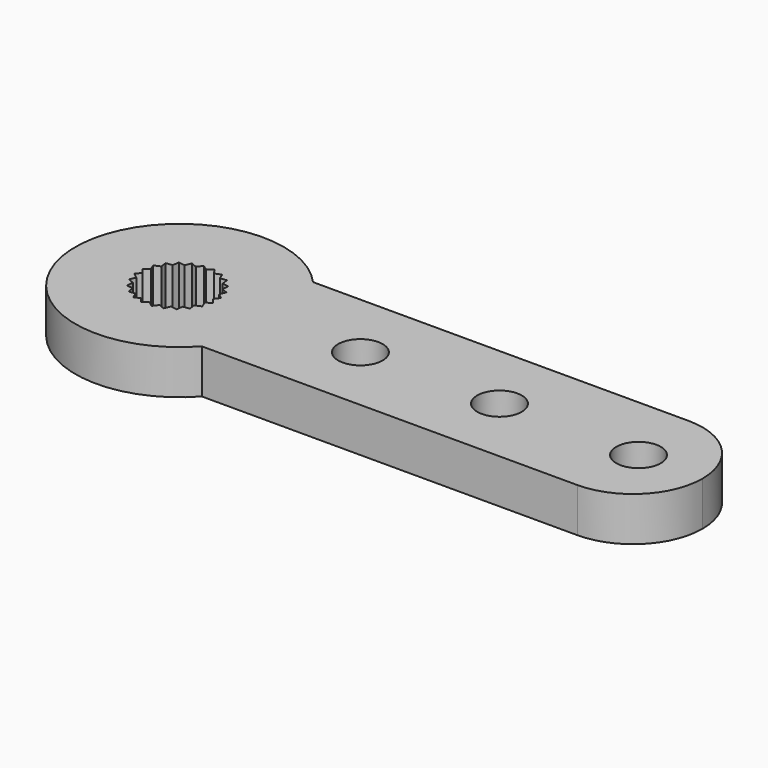
from build123d import *

# Parameters (mm, degrees)
F0_R     = 1.6
F1_DEPTH = 3.175


# Not quite as in the source:
# - a feature names something its author has since deleted; it is built from what else it names


with BuildPart() as f1:
    # F0 (on Top) → F1 (new body)
    with BuildSketch(Plane.XY):
        with BuildLine():
            Line((32.6, 5), (5.5901699437, 5))
            ThreePointArc((5.5901699437, 5), (-7.5, 0), (5.5901699437, -5))
            Line((5.5901699437, -5), (32.6, -5))
            ThreePointArc((32.6, -5), (36.1355339059, -3.5355339059), (37.6, 0))
            ThreePointArc((37.6, 0), (36.1355339059, 3.5355339059), (32.6, 5))
        make_face()
        Polygon((-0.4246363361, 2.7189872831), (-0.0526366882, 2.4335419138), (0.3193629596, 2.7189872831), (0.6048083289, 2.3469876353), (1.038011094, 2.5264260959), (1.2174495546, 2.0932233308), (1.6823333844, 2.154426448), (1.7435365017, 1.6895426182), (2.2084203316, 1.6283395009), (2.1472172143, 1.163455671), (2.5804199794, 0.9840172105), (2.4009815188, 0.5508144453), (2.7729811667, 0.265369076), (2.4875357974, -0.1066305718), (2.7729811667, -0.4786302196), (2.4009815188, -0.7640755889), (2.5804199794, -1.197278354), (2.1472172143, -1.3767168146), (2.2084203316, -1.8416006445), (1.7435365017, -1.9028037618), (1.6823333844, -2.3676875916), (1.2174495546, -2.3064844743), (1.038011094, -2.7396872394), (0.6048083289, -2.5602487789), (0.3193629596, -2.9322484267), (-0.0526366882, -2.6468030574), (-0.4246363361, -2.9322484267), (-0.7100817054, -2.5602487789), (-1.1432844705, -2.7396872394), (-1.322722931, -2.3064844743), (-1.7876067609, -2.3676875916), (-1.8488098782, -1.9028037618), (-2.3136937081, -1.8416006445), (-2.2524905908, -1.3767168146), (-2.6856933559, -1.197278354), (-2.5062548953, -0.7640755889), (-2.8782545432, -0.4786302196), (-2.5928091739, -0.1066305718), (-2.8782545432, 0.265369076), (-2.5062548953, 0.5508144453), (-2.6856933559, 0.9840172105), (-2.2524905908, 1.163455671), (-2.3136937081, 1.6283395009), (-1.8488098782, 1.6895426182), (-1.7876067609, 2.154426448), (-1.322722931, 2.0932233308), (-1.1432844705, 2.5264260959), (-0.7100817054, 2.3469876353), align=None, mode=Mode.SUBTRACT)
        with Locations((13, 0)):
            Circle(F0_R, mode=Mode.SUBTRACT)
        with Locations((23, 0)):
            Circle(F0_R, mode=Mode.SUBTRACT)
        with Locations((33, 0)):
            Circle(F0_R, mode=Mode.SUBTRACT)
    extrude(amount=F1_DEPTH)


solid = f1.part
